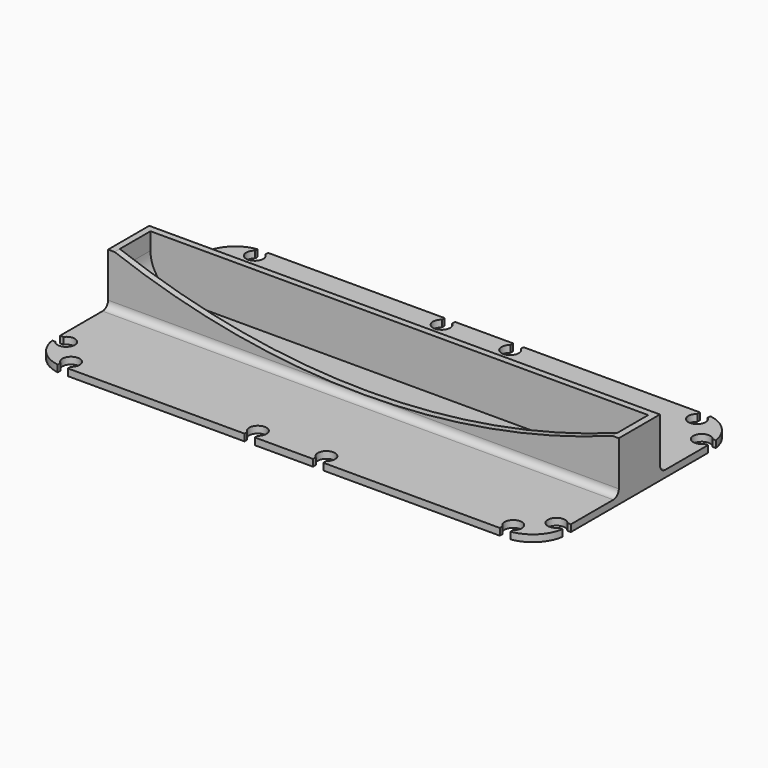
from build123d import *

# Parameters (mm, degrees)
F1_DEPTH     = 2
F2_W         = 149
F2_H         = 15
F3_DEPTH     = 15
F4_W         = 145.2
F4_H         = 11.2
F5_DEPTH     = 15
F7_DEPTH     = 13.1
F8_TEXT_SIZE = 13.8888888889
F9_DEPTH     = 0.5
F10_R        = 1.99999
F11_T1_DEPTH = 11.2
F11_T3_DEPTH = 51.4342998332


# Not quite as in the source:
# - a fillet or chamfer that OpenCascade refuses, or shapes differently, is made with other operations: its cross-section is extruded or revolved along the edge and cut away or added
# - a fillet or chamfer is up to 0.001 mm smaller than in the source, because OpenCascade refuses the exact size
# - Text() gives the source's letters only with a copy of the font that has no kerning and outlines rounded to 1/6400 em; it was checked with that copy


with BuildPart() as f1:
    # F0 (on Top) → F1 (new body)
    with BuildSketch(Plane.XY):
        with BuildLine():
            Line((66, -36.5), (74.5, -36.5))
            Line((74.5, -36.5), (74.5, -28))
            Line((74.5, -28), (73.5, -28))
            ThreePointArc((73.5, -28), (69, -26.5), (73.5, -25))
            Line((73.5, -25), (74.5, -25))
            Line((74.5, -25), (74.5, 25))
            Line((74.5, 25), (73.5, 25))
            ThreePointArc((73.5, 25), (69, 26.5), (73.5, 28))
            Line((73.5, 28), (74.5, 28))
            Line((74.5, 28), (74.5, 36.5))
            Line((74.5, 36.5), (66, 36.5))
            Line((66, 36.5), (66, 35.5))
            ThreePointArc((66, 35.5), (64.5, 31), (63, 35.5))
            Line((63, 35.5), (63, 36.5))
            Line((63, 36.5), (11.5, 36.5))
            Line((11.5, 36.5), (11.5, 35.5))
            ThreePointArc((11.5, 35.5), (10, 31), (8.5, 35.5))
            Line((8.5, 35.5), (8.5, 36.5))
            Line((8.5, 36.5), (-8.5, 36.5))
            Line((-8.5, 36.5), (-8.5, 35.5))
            ThreePointArc((-8.5, 35.5), (-10, 31), (-11.5, 35.5))
            Line((-11.5, 35.5), (-11.5, 36.5))
            Line((-11.5, 36.5), (-63, 36.5))
            Line((-63, 36.5), (-63, 35.5))
            ThreePointArc((-63, 35.5), (-64.5, 31), (-66, 35.5))
            Line((-66, 35.5), (-66, 36.5))
            Line((-66, 36.5), (-74.5, 36.5))
            Line((-74.5, 36.5), (-74.5, 28))
            Line((-74.5, 28), (-73.5, 28))
            ThreePointArc((-73.5, 28), (-69, 26.5), (-73.5, 25))
            Line((-73.5, 25), (-74.5, 25))
            Line((-74.5, 25), (-74.5, -25))
            Line((-74.5, -25), (-73.5, -25))
            ThreePointArc((-73.5, -25), (-69, -26.5), (-73.5, -28))
            Line((-73.5, -28), (-74.5, -28))
            Line((-74.5, -28), (-74.5, -36.5))
            Line((-74.5, -36.5), (-66, -36.5))
            Line((-66, -36.5), (-66, -35.5))
            ThreePointArc((-66, -35.5), (-64.5, -31), (-63, -35.5))
            Line((-63, -35.5), (-63, -36.5))
            Line((-63, -36.5), (-11.5, -36.5))
            Line((-11.5, -36.5), (-11.5, -35.5))
            ThreePointArc((-11.5, -35.5), (-10, -31), (-8.5, -35.5))
            Line((-8.5, -35.5), (-8.5, -36.5))
            Line((-8.5, -36.5), (8.5, -36.5))
            Line((8.5, -36.5), (8.5, -35.5))
            ThreePointArc((8.5, -35.5), (10, -31), (11.5, -35.5))
            Line((11.5, -35.5), (11.5, -36.5))
            Line((11.5, -36.5), (63, -36.5))
            Line((63, -36.5), (63, -35.5))
            ThreePointArc((63, -35.5), (64.5, -31), (66, -35.5))
            Line((66, -35.5), (66, -36.5))
        make_face()
    extrude(amount=F1_DEPTH)

    # F2 (on face) → F3 (join)
    with BuildSketch(Plane.XY.offset(2)):
        Rectangle(F2_W, F2_H)
    extrude(amount=F3_DEPTH)

    # F4 (on face) → F5 (cut, through all)
    with BuildSketch(Plane.XY.offset(17)):
        Rectangle(F4_W, F4_H)
    extrude(amount=-F5_DEPTH, mode=Mode.SUBTRACT)

    # F6 (on face) → F7 (cut, through all)
    with BuildSketch(Plane.XZ.offset(7.5)):
        with BuildLine():
            Line((72.6, 17), (-72.6, 17))
            ThreePointArc((-72.6, 17), (0, 4), (72.6, 17))
        make_face()
    extrude(amount=-F7_DEPTH, mode=Mode.SUBTRACT)

    # F8 (on face) → F9 (join)
    with BuildSketch(Plane(origin=(0, 7.5, 0), x_dir=(-1, 0, 0), z_dir=(0, 1, 0))):
        with Locations((-11.8934461806, 4.5)):
            Text('3E8', F8_TEXT_SIZE, font='Open Sans', text_align=(TextAlign.LEFT, TextAlign.BOTTOM))
    extrude(amount=F9_DEPTH)

    # F10 (radius 2 in the source; OpenCascade refuses exactly that, so slightly less here)
    f10_edges = [f1.edges().sort_by_distance(p)[0] for p in [
        (0, -7.5, 2),
        (0, 7.5, 2),
    ]]
    fillet(f10_edges, radius=F10_R)

    # F11: fillet of radius 10 on 6 edges, made by hand

    # F11_s2 → F11_t1 (join)
    with BuildSketch(Plane.XZ.offset(-5.6)):
        with BuildLine():
            ThreePointArc((-72.6, 12), (-69.6710678119, 4.9289321881), (-62.6, 2))
            Line((-62.6, 2), (-72.6, 2))
            Line((-72.6, 2), (-72.6, 12))
        make_face()
        with BuildLine():
            ThreePointArc((72.6, 12), (69.6710678119, 4.9289321881), (62.6, 2))
            Line((62.6, 2), (72.6, 2))
            Line((72.6, 2), (72.6, 12))
        make_face()
    extrude(amount=F11_T1_DEPTH)

    # F11_s4 → F11_t3 (cut)
    with BuildSketch(Plane.XY.offset(-24.7171499166)):
        with BuildLine():
            ThreePointArc((74.5, -28), (71.1323424386, -34.0828754441), (64.6131400334, -36.5))
            Line((64.6131400334, -36.5), (74.5, -36.5))
            Line((74.5, -36.5), (74.5, -28))
        make_face()
        with BuildLine():
            ThreePointArc((74.5, 26.6131400334), (72.0828754441, 33.1323424386), (66, 36.5))
            Line((66, 36.5), (74.5, 36.5))
            Line((74.5, 36.5), (74.5, 26.6131400334))
        make_face()
        with BuildLine():
            ThreePointArc((-74.5, -26.6131400334), (-72.0828754441, -33.1323424386), (-66, -36.5))
            Line((-66, -36.5), (-74.5, -36.5))
            Line((-74.5, -36.5), (-74.5, -26.6131400334))
        make_face()
        with BuildLine():
            ThreePointArc((-74.5, 28), (-71.1323424386, 34.0828754441), (-64.6131400334, 36.5))
            Line((-64.6131400334, 36.5), (-74.5, 36.5))
            Line((-74.5, 36.5), (-74.5, 28))
        make_face()
    extrude(amount=F11_T3_DEPTH, mode=Mode.SUBTRACT)


solid = f1.part
